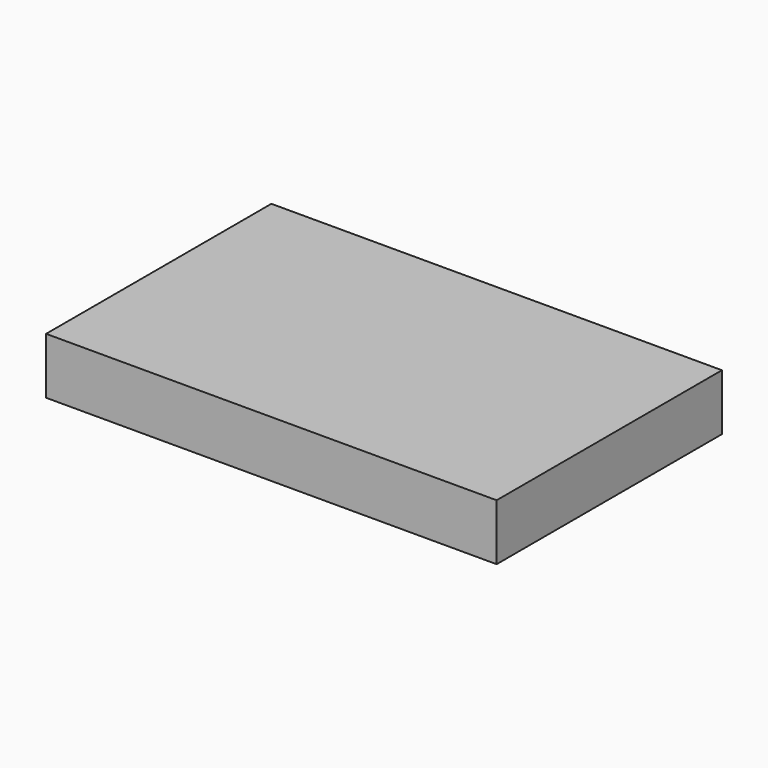
from build123d import *

# Parameters (mm, degrees)
F0_W           = 101.6
F0_H           = 63.5
F1_DEPTH       = 12.7
F2_T           = -4.7625
F3_TEXT_SIZE   = 6.6322222222
F3_TEXT_SIZE_2 = 6.6322183895
F4_DEPTH       = 0.635


# Not quite as in the source:
# - Text() gives the source's letters only with a copy of the font that has no kerning and outlines rounded to 1/6400 em; it was checked with that copy


with BuildPart() as f1:
    # F0 (on Top) → F1 (new body)
    with BuildSketch(Plane.XY):
        Rectangle(F0_W, F0_H)
    extrude(amount=F1_DEPTH)

    # F2
    f2_openings = [f1.faces().sort_by_distance(p)[0] for p in [
        (0, 0, 0),
    ]]
    offset(amount=F2_T, openings=f2_openings)

    # F3 (on face) → F4 (join)
    with BuildSketch(Plane(origin=(0, 0, 7.9375), x_dir=(1, 0, 0), z_dir=(0, 0, -1))):
        with Locations((-44.5084616273, -25.3487718902)):
            Text('for idalmy', F3_TEXT_SIZE, font='Open Sans', font_style=FontStyle.ITALIC, text_align=(TextAlign.LEFT, TextAlign.BOTTOM))
        with Locations((30.82883161, -25.3487718902)):
            Text('2.17', F3_TEXT_SIZE_2, font='Open Sans', font_style=FontStyle.ITALIC, text_align=(TextAlign.LEFT, TextAlign.BOTTOM))
    extrude(amount=F4_DEPTH)


solid = f1.part
